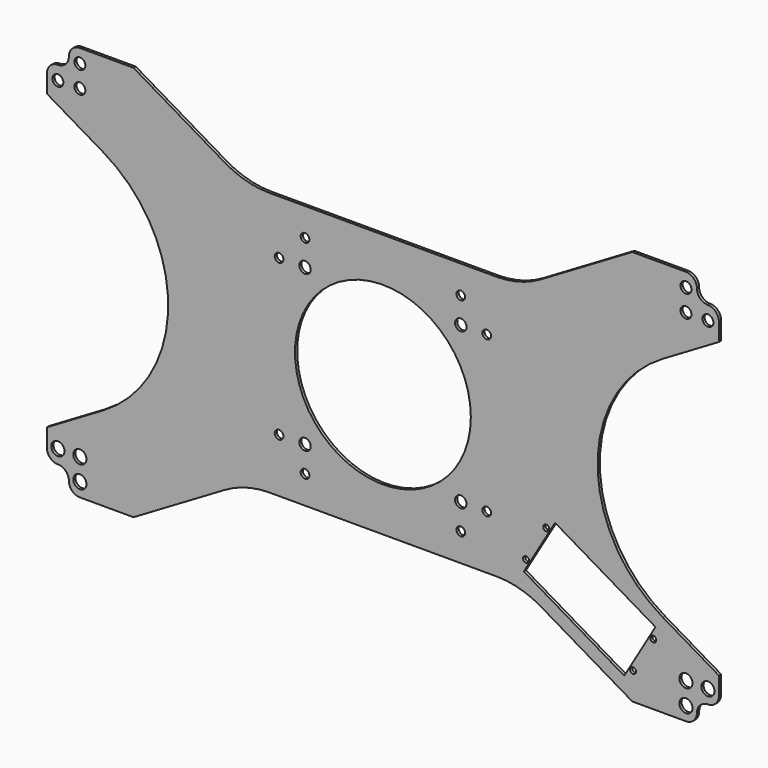
from build123d import *

# Parameters (mm, degrees)
F0_R     = 3.81
F0_R_2   = 2.5
F0_R_3   = 3.3
F0_R_4   = 1.72466
F0_R_5   = 3.175
F0_R_6   = 50.8
F1_DEPTH = 1.5875
F2_R     = 6.34999


# Not quite as in the source:
# - a fillet or chamfer is up to 0.001 mm smaller than in the source, because OpenCascade refuses the exact size


with BuildPart() as f1:
    # F0 (on Front) → F1 (new body)
    with BuildSketch(Plane.XZ):
        with BuildLine():
            Line((-6.35, 207.9625), (-19.05, 207.9625))
            Line((-19.05, 207.9625), (-19.05, 191.187323006))
            Line((-19.05, 191.187323006), (13.4939129862, 172.0272456399))
            ThreePointArc((13.4939129862, 172.0272456399), (51.0340994838, 106.3625), (13.4939129862, 40.6977543601))
            Line((13.4939129862, 40.6977543601), (-19.05, 21.537676994))
            Line((-19.05, 21.537676994), (-19.05, 4.7625))
            Line((-19.05, 4.7625), (-6.35, 4.7625))
            Line((-6.35, 4.7625), (-6.35, -7.9375))
            Line((-6.35, -7.9375), (31.0143905041, -7.9375))
            Line((31.0143905041, -7.9375), (83.7986667883, 23.1389970933))
            ThreePointArc((83.7986667883, 23.1389970933), (96.215342788, 28.3751822993), (109.5718757899, 30.1625))
            Line((109.5718757899, 30.1625), (240.6114472101, 30.1625))
            ThreePointArc((240.6114472101, 30.1625), (253.967980212, 28.3751822993), (266.3846562117, 23.1389970933))
            Line((266.3846562117, 23.1389970933), (319.1689324959, -7.9375))
            Line((319.1689324959, -7.9375), (356.533323, -7.9375))
            Line((356.533323, -7.9375), (356.533323, 4.7625))
            Line((356.533323, 4.7625), (369.233323, 4.7625))
            Line((369.233323, 4.7625), (369.233323, 21.537676994))
            Line((369.233323, 21.537676994), (336.6894100138, 40.6977543601))
            ThreePointArc((336.6894100138, 40.6977543601), (299.1492235162, 106.3625), (336.6894100138, 172.0272456399))
            Line((336.6894100138, 172.0272456399), (369.233323, 191.187323006))
            Line((369.233323, 191.187323006), (369.233323, 207.9625))
            Line((369.233323, 207.9625), (356.533323, 207.9625))
            Line((356.533323, 207.9625), (356.533323, 220.6625))
            Line((356.533323, 220.6625), (319.1689324959, 220.6625))
            Line((319.1689324959, 220.6625), (266.3846562117, 189.5860029067))
            ThreePointArc((266.3846562117, 189.5860029067), (253.967980212, 184.3498177007), (240.6114472101, 182.5625))
            Line((240.6114472101, 182.5625), (109.5718757899, 182.5625))
            ThreePointArc((109.5718757899, 182.5625), (96.215342788, 184.3498177007), (83.7986667883, 189.5860029067))
            Line((83.7986667883, 189.5860029067), (31.0143905041, 220.6625))
            Line((31.0143905041, 220.6625), (-6.35, 220.6625))
            Line((-6.35, 220.6625), (-6.35, 207.9625))
        make_face()
        Circle(F0_R, mode=Mode.SUBTRACT)
        with Locations((-12.7, 12.7)):
            Circle(F0_R, mode=Mode.SUBTRACT)
        with Locations((0, 12.7)):
            Circle(F0_R, mode=Mode.SUBTRACT)
        with Locations((130.0916615, 46.3625)):
            Circle(F0_R_2, mode=Mode.SUBTRACT)
        with Locations((115.0916615, 61.3625)):
            Circle(F0_R_2, mode=Mode.SUBTRACT)
        with Locations((130.0916615, 61.3625)):
            Circle(F0_R_3, mode=Mode.SUBTRACT)
        with Locations((220.0916615, 46.3625)):
            Circle(F0_R_2, mode=Mode.SUBTRACT)
        with Locations((257.7919761398, 44.3280112686)):
            Circle(F0_R_4, mode=Mode.SUBTRACT)
        with Locations((319.6223383993, 7.9256731426)):
            Circle(F0_R_4, mode=Mode.SUBTRACT)
        with Locations((350.183323, 0)):
            Circle(F0_R, mode=Mode.SUBTRACT)
        with Locations((350.183323, 12.7)):
            Circle(F0_R, mode=Mode.SUBTRACT)
        with Locations((362.883323, 12.7)):
            Circle(F0_R, mode=Mode.SUBTRACT)
        Polygon((314.5229509507, 3.6403531184), (256.5190923021, 37.7898550455), (274.5603386032, 68.4334030108), (332.5641972518, 34.2839010837), align=None, mode=Mode.SUBTRACT)
        with Locations((331.2913134141, 27.7457448606)):
            Circle(F0_R_4, mode=Mode.SUBTRACT)
        with Locations((220.0916615, 61.3625)):
            Circle(F0_R_3, mode=Mode.SUBTRACT)
        with Locations((235.0916615, 61.3625)):
            Circle(F0_R_2, mode=Mode.SUBTRACT)
        with Locations((269.4609511546, 64.1480829866)):
            Circle(F0_R_4, mode=Mode.SUBTRACT)
        with Locations((115.0916615, 151.3625)):
            Circle(F0_R_2, mode=Mode.SUBTRACT)
        with Locations((130.0916615, 151.3625)):
            Circle(F0_R_3, mode=Mode.SUBTRACT)
        with Locations((-12.7, 200.025)):
            Circle(F0_R_5, mode=Mode.SUBTRACT)
        with Locations((0, 200.025)):
            Circle(F0_R_5, mode=Mode.SUBTRACT)
        with Locations((0, 212.725)):
            Circle(F0_R_5, mode=Mode.SUBTRACT)
        with Locations((130.0916615, 166.3625)):
            Circle(F0_R_2, mode=Mode.SUBTRACT)
        with Locations((175.0916615, 106.3625)):
            Circle(F0_R_6, mode=Mode.SUBTRACT)
        with Locations((220.0916615, 151.3625)):
            Circle(F0_R_3, mode=Mode.SUBTRACT)
        with Locations((235.0916615, 151.3625)):
            Circle(F0_R_2, mode=Mode.SUBTRACT)
        with Locations((220.0916615, 166.3625)):
            Circle(F0_R_2, mode=Mode.SUBTRACT)
        with Locations((350.183323, 200.025)):
            Circle(F0_R_5, mode=Mode.SUBTRACT)
        with Locations((362.883323, 200.025)):
            Circle(F0_R_5, mode=Mode.SUBTRACT)
        with Locations((350.183323, 212.725)):
            Circle(F0_R_5, mode=Mode.SUBTRACT)
    extrude(amount=F1_DEPTH)

    # F2 (radius 6.35 in the source; OpenCascade refuses exactly that, so slightly less here)
    f2_edges = [f1.edges().sort_by_distance(p)[0] for p in [
        (-6.35, -0.79375, 207.9625),
        (-6.35, -0.79375, 220.6625),
        (-19.05, -0.79375, 207.9625),
        (356.533323, -0.79375, 207.9625),
        (356.533323, -0.79375, 220.6625),
        (369.233323, -0.79375, 207.9625),
        (356.533323, -0.79375, 4.7625),
        (369.233323, -0.79375, 4.7625),
        (356.533323, -0.79375, -7.9375),
        (-6.35, -0.79375, 4.7625),
        (-19.05, -0.79375, 4.7625),
        (-6.35, -0.79375, -7.9375),
    ]]
    fillet(f2_edges, radius=F2_R)


solid = f1.part
